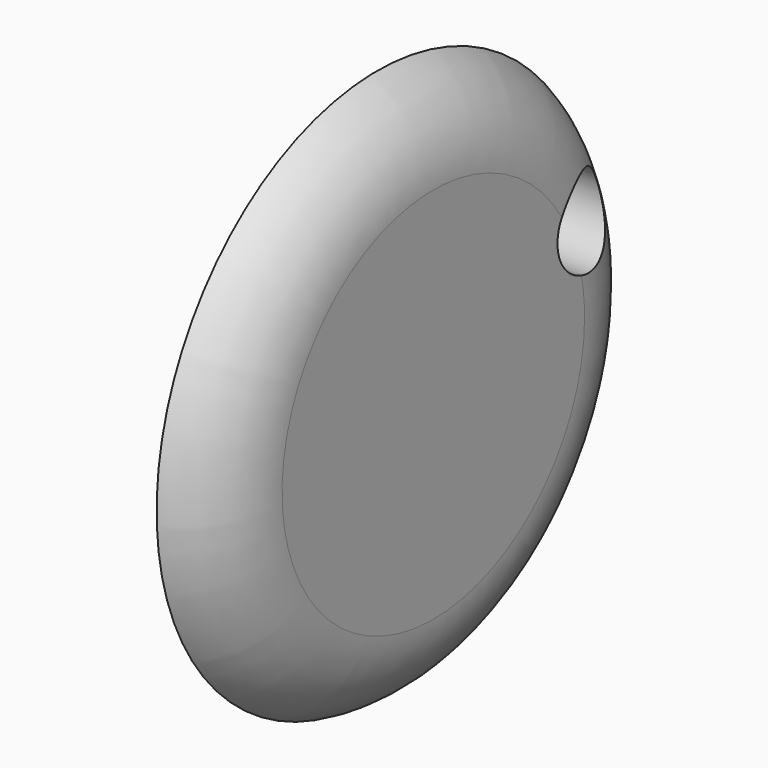
from build123d import *

# Parameters (mm, degrees)
F0_R     = 149.022421697
F0_R_2   = 22.7529674453
F1_DEPTH = 30.3589943796


# Not quite as in the source:
# - a fillet or chamfer that OpenCascade refuses, or shapes differently, is made with other operations: its cross-section is extruded or revolved along the edge and cut away or added


with BuildPart() as f1:
    # F0 (on Right) → F1 (new body)
    with BuildSketch(Plane.YZ):
        with Locations((15.6553536654, -18.1811377406)):
            Circle(F0_R)
        with Locations((122.302301228, 24.3675112724)):
            Circle(F0_R_2, mode=Mode.SUBTRACT)
    extrude(amount=F1_DEPTH)

    # F2: fillet of radius 51.2848670586 on 1 edges, made by hand

    # F2_s1 → F2_t2 (revolve, cut)
    with BuildSketch(Plane.XY.offset(-18.1811377406)):
        with BuildLine():
            ThreePointArc((0, 164.6777753623), (22.105035908, 145.7575820929), (30.3589943796, 117.8563546038))
            Line((30.3589943796, 117.8563546038), (30.3589943796, 164.6777753623))
            Line((30.3589943796, 164.6777753623), (0, 164.6777753623))
        make_face()
    revolve(axis=Axis((30.3589943796, 15.6553536654, -18.1811377406), (1, 0, 0)), mode=Mode.SUBTRACT)


solid = f1.part
